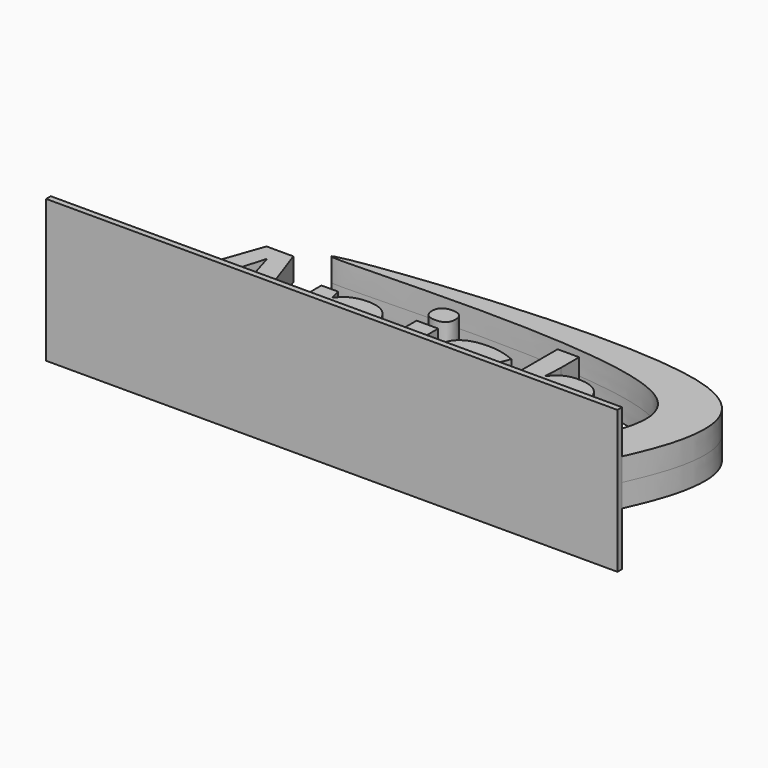
from build123d import *

# Parameters (mm, degrees)
F0_TEXT_SIZE = 160.5737333496
F1_DEPTH     = 25.4
F2_W         = 633.317142725
F2_H         = 157.9945459962
F3_DEPTH     = 6.45792
F5_DEPTH     = 25.4


# Not quite as in the source:
# - Text() gives the source's letters only with a copy of the font that has no kerning and outlines rounded to 1/6400 em; it was checked with that copy


with BuildPart() as f1:
    # F0 (on Top) → F1 (new body)
    with BuildSketch(Plane.XY):
        with Locations((-208.3814591169, -90.8005982637)):
            Text('Anish', F0_TEXT_SIZE, font='Open Sans', font_style=FontStyle.BOLD, text_align=(TextAlign.LEFT, TextAlign.BOTTOM))
    extrude(amount=F1_DEPTH)


with BuildPart() as f3:
    # F2 (on face) → F3 (new body)
    with BuildSketch(Plane.XZ.offset(90.8005982637)):
        with Locations((1.6856640577, -5.6110359728)):
            Rectangle(F2_W, F2_H)
    extrude(amount=F3_DEPTH)

    # F4 (on Top) → F5 (join, symmetric)
    with BuildSketch(Plane.XY):
        with BuildLine():
            add(Edge.make_bspline(
                [(267.5442354202, -90.8005982637), (290.7893265047, -47.1923836603), (337.1490496756, 77.2058694118), (-404.8001610137, 12.6981954817), (323.6602296754, 109.9598441214), (350.756497966, -16.3102938407), (328.3738246788, -68.0746418356), (318.3442354202, -90.8005982637)],
                knots=[0, 0, 0, 0, 0.1540647576, 0.4373432798, 0.7290768982, 0.871325167, 1, 1, 1, 1], degree=3))
            Line((267.5442354202, -90.8005982637), (318.3442354202, -90.8005982637))
        make_face()
    extrude(amount=F5_DEPTH, both=True)


solid = Compound([f1.part, f3.part])
